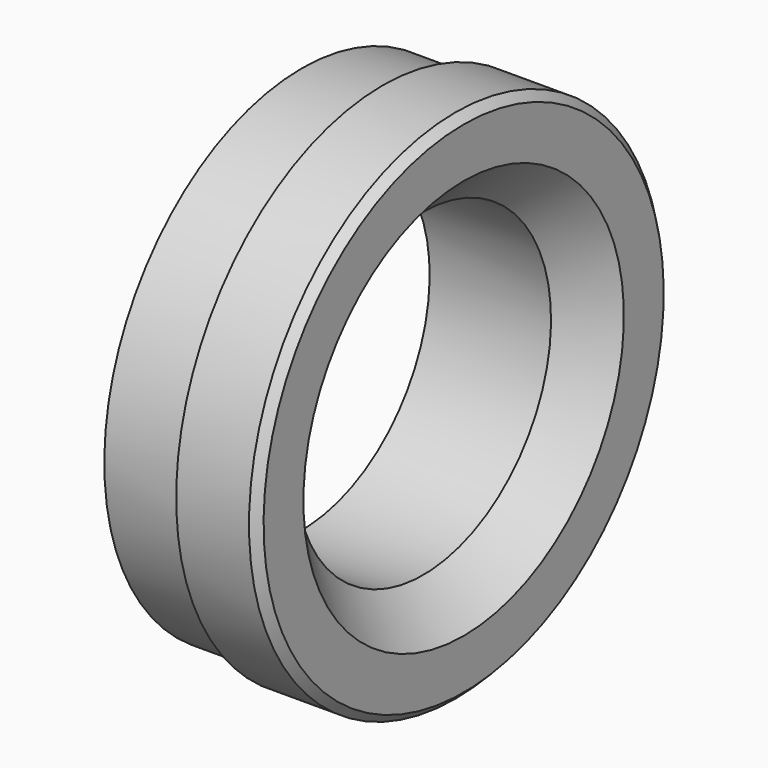
from build123d import *

# Parameters (mm, degrees)
F2_SIZE      = 1
F3_SIZE      = 5
F4_TEXT_SIZE = 8.7792598541
F5_DEPTH     = 0.5


# Not quite as in the source:
# - Text() gives the source's letters only with a copy of the font that has no kerning and outlines rounded to 1/6400 em; it was checked with that copy


with BuildPart() as f1:
    # F0 (on Front) → F1 (revolve)
    with BuildSketch(Plane.XZ):
        Polygon((0, 30.5), (0, 19.75), (20, 19.75), (20, 31.9), (10, 31.9), (10, 30.5), align=None)
    revolve(axis=Axis((22.5499981313, 0, 0), (1, 0, 0)))

    # F2
    f2_edges = [f1.edges().sort_by_distance(p)[0] for p in [
        (20, 0, -31.9),
    ]]
    chamfer(f2_edges, length=F2_SIZE)

    # F3
    f3_edges = [f1.edges().sort_by_distance(p)[0] for p in [
        (20, 0, -19.75),
    ]]
    chamfer(f3_edges, length=F3_SIZE)

    # F4 (on face) → F5 (cut)
    with BuildSketch(Plane(origin=(0, 0, 0), x_dir=(0, -1, 0), z_dir=(-1, 0, 0))):
        with Locations((-8.7291906378, 21.4875378719)):
            Text('39.5', F4_TEXT_SIZE, font='Open Sans', text_align=(TextAlign.LEFT, TextAlign.BOTTOM))
    extrude(amount=-F5_DEPTH, mode=Mode.SUBTRACT)


solid = f1.part
